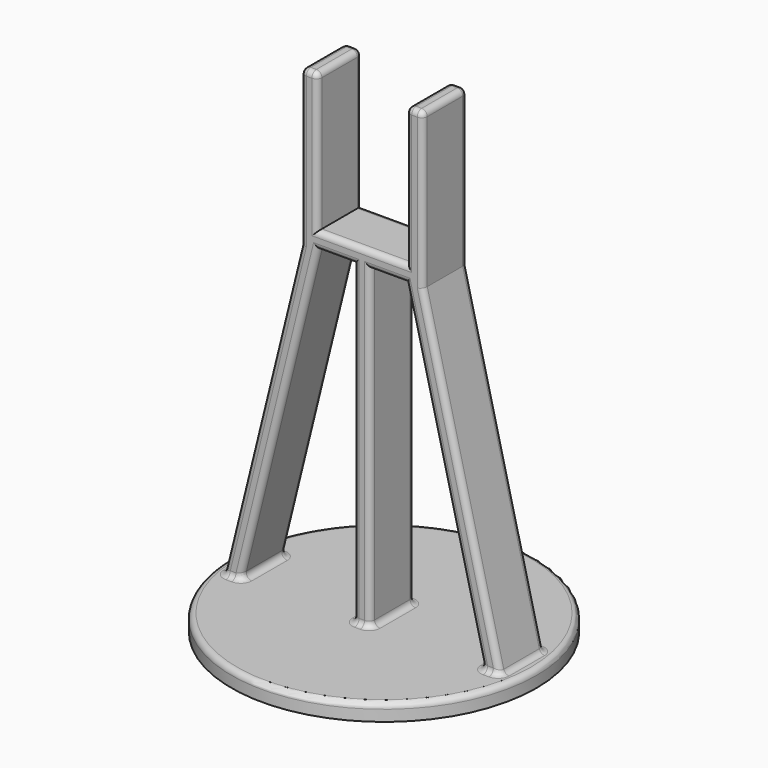
from build123d import *

# Parameters (mm, degrees)
F1_DEPTH = 10
F3_DEPTH = 25
F4_R     = 27.495097568
F5_DEPTH = 3
F6_R     = 1


# Not quite as in the source:
# - a feature names something its author has since deleted; it is built from what else it names


with BuildPart() as f1:
    # F0 (on Front) → F1 (new body)
    with BuildSketch(Plane.XZ):
        Polygon((11, 12.5), (8, 12.5), (8, -12.5), (-8, -12.5), (-8, 12.5), (-11, 12.5), (-11, -15.5), (11, -15.5), align=None)
        Polygon((25, -72.5), (11, -15.5), (-11, -15.5), (-25, -72.5), align=None)
    extrude(amount=F1_DEPTH)

    # F2 (on face) → F3 (cut)
    with BuildSketch(Plane.XZ.offset(10)):
        Polygon((-1.5, -15.5), (-7.9108356651, -15.5), (-21.9108356651, -72.5), (-1.5, -72.5), align=None)
        Polygon((1.5, -15.5), (1.5, -72.5), (21.9108356651, -72.5), (7.9108356651, -15.5), align=None)
    extrude(amount=-F3_DEPTH, mode=Mode.SUBTRACT)

    # F4 (on face) → F5 (join)
    with BuildSketch(Plane(origin=(0, 0, -72.5), x_dir=(1, 0, 0), z_dir=(0, 0, -1))):
        with Locations((0, 5)):
            Circle(F4_R)
    extrude(amount=F5_DEPTH)

    # F6
    f6_edges = [f1.edges().sort_by_distance(p)[0] for p in [
        (-8, -5, 12.5),
        (8, -5, 12.5),
        (11, -5, 12.5),
        (-11, -5, 12.5),
        (9.5, -10, 12.5),
        (-9.5, -10, 12.5),
        (9.5, 0, 12.5),
        (-9.5, 0, 12.5),
        (-11, 0, -1.5),
        (11, 0, -1.5),
        (11, -10, -1.5),
        (-11, -10, -1.5),
        (-18, -10, -44),
        (18, -10, -44),
        (-18, 0, -44),
        (18, 0, -44),
        (0, -10, -72.5),
        (23.455418, -10, -72.5),
        (14.910836, -10, -44),
        (4.705418, -10, -15.5),
        (1.5, -10, -44),
        (-1.5, -10, -44),
        (-4.705418, -10, -15.5),
        (-14.910836, -10, -44),
        (-23.455418, -10, -72.5),
        (-8, -10, 0),
        (0, -10, -12.5),
        (8, -10, 0),
        (23.455418, 0, -72.5),
        (14.910836, 0, -44),
        (4.705418, 0, -15.5),
        (1.5, 0, -44),
        (0, 0, -72.5),
        (-1.5, 0, -44),
        (-4.705418, 0, -15.5),
        (-14.910836, 0, -44),
        (-23.455418, 0, -72.5),
        (-8, 0, 0),
        (0, 0, -12.5),
        (8, 0, 0),
        (-27.495098, -5, -72.5),
        (-21.910836, -5, -72.5),
        (-25, -5, -72.5),
        (1.5, -5, -72.5),
        (-1.5, -5, -72.5),
        (25, -5, -72.5),
        (21.910836, -5, -72.5),
    ]]
    fillet(f6_edges, radius=F6_R)


solid = f1.part
